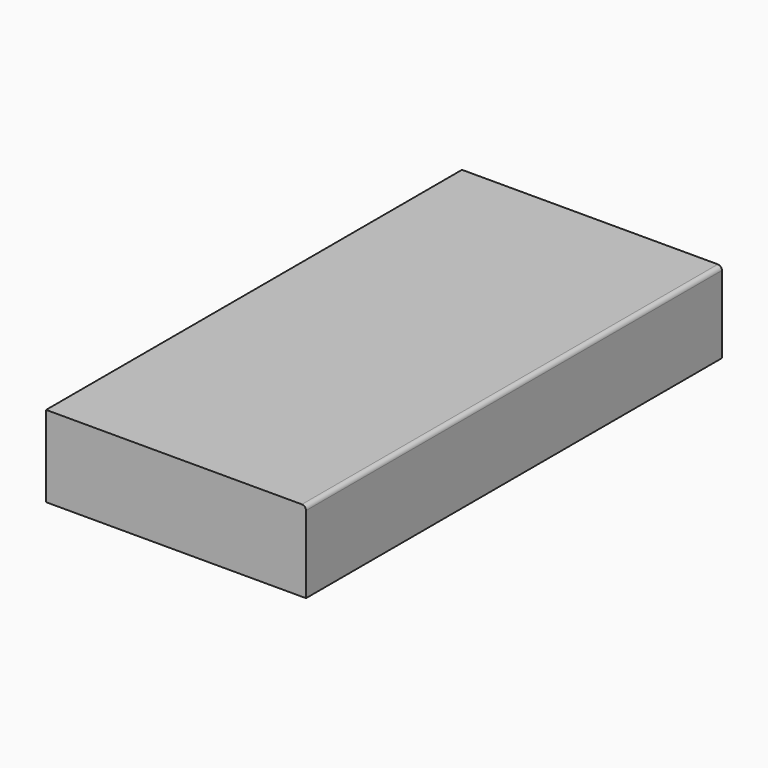
from build123d import *

# Parameters (mm, degrees)
F0_W     = 16.002
F0_H     = 32.004
F1_DEPTH = 5.0038
F4_R     = 0.254


# Not quite as in the source:
# - the program builds the solid bodies; features that only make, move or delete a surface that nothing else refers to are left out


with BuildPart() as f1:
    # F0 (on Top) → F1 (new body)
    with BuildSketch(Plane.XY):
        with Locations((-18.6587861177, 4.6874228865)):
            Rectangle(F0_W, F0_H)
    extrude(amount=F1_DEPTH)

    # F4
    f4_edges = [f1.edges().sort_by_distance(p)[0] for p in [
        (-10.657786, 4.687423, 5.0038),
    ]]
    fillet(f4_edges, radius=F4_R)


solid = f1.part
